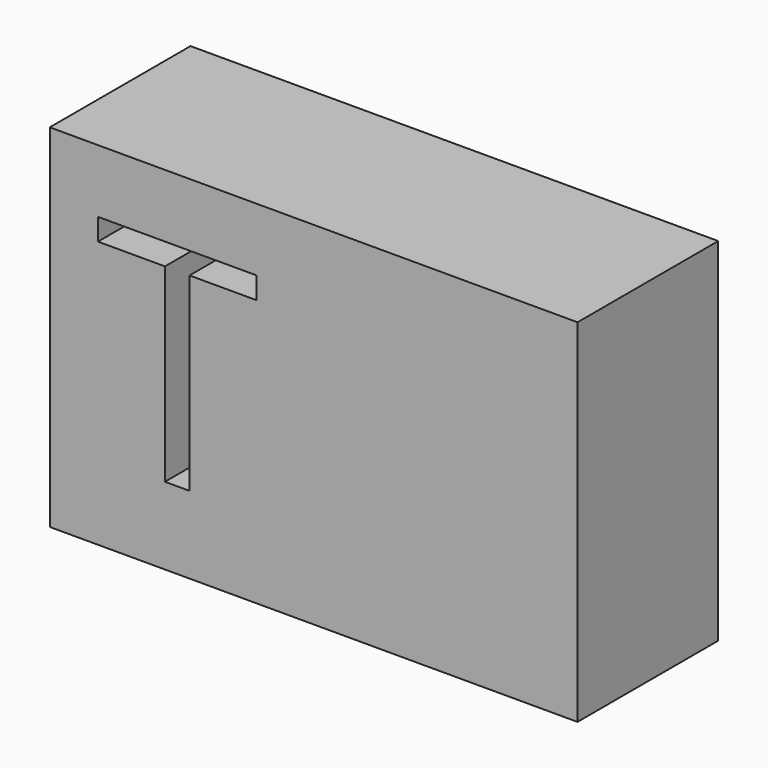
from build123d import *

# Parameters (mm, degrees)
F0_W         = 76.2
F0_H         = 50.8
F1_DEPTH     = 25.4
F2_TEXT_SIZE = 42.7711328181
F3_DEPTH     = 12.7


# Not quite as in the source:
# - Text() gives the source's letters only with a copy of the font that has no kerning and outlines rounded to 1/6400 em; it was checked with that copy


with BuildPart() as f1:
    # F0 (on Front) → F1 (new body)
    with BuildSketch(Plane.XZ):
        Rectangle(F0_W, F0_H)
    extrude(amount=F1_DEPTH)

    # F2 (on face) → F3 (cut)
    with BuildSketch(Plane.XZ.offset(25.4)):
        with Locations((-31.5147303045, -14.2463846132)):
            Text('T', F2_TEXT_SIZE, font='Open Sans', text_align=(TextAlign.LEFT, TextAlign.BOTTOM))
    extrude(amount=-F3_DEPTH, mode=Mode.SUBTRACT)


solid = f1.part
